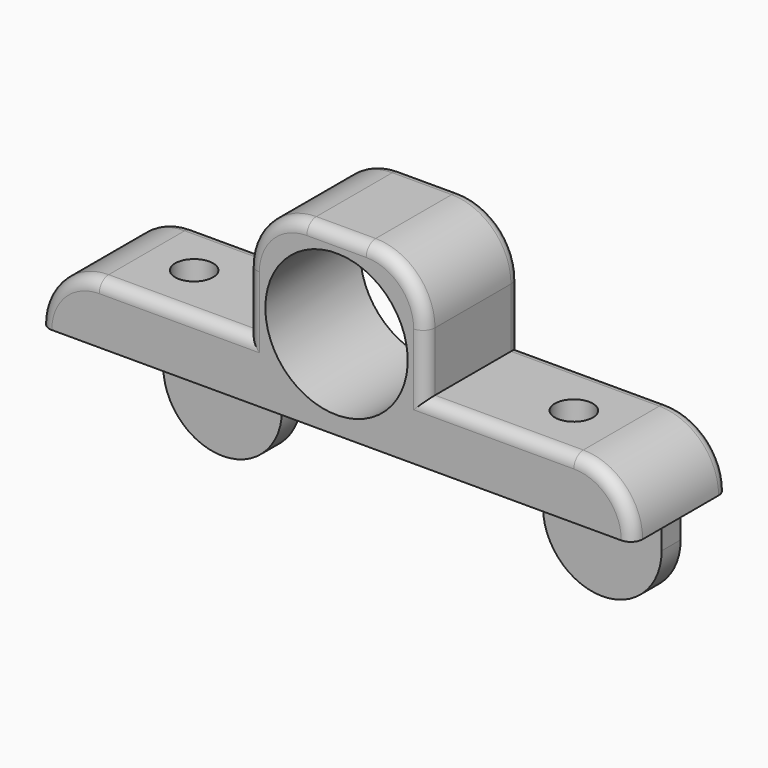
from build123d import *

# Parameters (mm, degrees)
F0_W         = 50
F0_H         = 10
F0_R         = 1.6
F1_DEPTH     = 5
F2_W         = 15
F2_H         = 10
F2_R         = 1.6
F3_DEPTH     = 10
F5_R         = 5
F6_R         = 4.99999
F4_R         = 6
F7_DEPTH     = 25
F8_T1_DEPTH  = 12.50001
F8_T3_DEPTH  = 5
F8_T5_DEPTH  = 5
F8_T7_DEPTH  = 12.50001
F8_T9_DEPTH  = 2.50001
F8_T12_ANGLE = 90
F8_T14_ANGLE = 90
F8_T16_ANGLE = 90
F8_T18_ANGLE = 90
F8_T20_ANGLE = 90
F8_T22_ANGLE = 90
F8_T24_ANGLE = 90
F8_T26_ANGLE = 90
F8_T31_DEPTH = 7.5
F8_T35_DEPTH = 15.00001
F8_T42_DEPTH = 15.00001
F8_T46_DEPTH = 7.5
F8_T53_DEPTH = 15.00001
F8_T57_DEPTH = 7.5
F8_T64_DEPTH = 7.5
F8_T68_DEPTH = 15.00001
F9_W         = 10
F9_H         = 2
F10_DEPTH    = 10
F11_R        = 4.99999


# Not quite as in the source:
# - a fillet or chamfer that OpenCascade refuses, or shapes differently, is made with other operations: its cross-section is extruded or revolved along the edge and cut away or added
# - a fillet or chamfer is up to 0.001 mm smaller than in the source, because OpenCascade refuses the exact size


with BuildPart() as f1:
    # F0 (on Top) → F1 (new body)
    with BuildSketch(Plane.XY):
        Rectangle(F0_W, F0_H)
        with Locations((-16, 0)):
            Circle(F0_R, mode=Mode.SUBTRACT)
        with Locations((16, 0)):
            Circle(F0_R, mode=Mode.SUBTRACT)
    extrude(amount=F1_DEPTH)

    # F2 (on face) → F3 (join)
    with BuildSketch(Plane.XY.offset(5)):
        Rectangle(F2_W, F2_H)
        with Locations((-3.9, 0)):
            Circle(F2_R, mode=Mode.SUBTRACT)
        with Locations((3.9, 0)):
            Circle(F2_R, mode=Mode.SUBTRACT)
        with Locations((3.9, 0)):
            Circle(F2_R)
        with Locations((-3.9, 0)):
            Circle(F2_R)
    extrude(amount=F3_DEPTH)

    # F5
    f5_edges = [f1.edges().sort_by_distance(p)[0] for p in [
        (7.5, 0, 15),
        (-7.5, 0, 15),
    ]]
    fillet(f5_edges, radius=F5_R)

    # F6 (radius 5 in the source; OpenCascade refuses exactly that, so slightly less here)
    f6_edges = [f1.edges().sort_by_distance(p)[0] for p in [
        (-25, 0, 5),
        (25, 0, 5),
    ]]
    fillet(f6_edges, radius=F6_R)

    # F4 (on face) → F7 (cut)
    with BuildSketch(Plane(origin=(0, 5, 0), x_dir=(-1, 0, 0), z_dir=(0, 1, 0))):
        with Locations((0, 7.5)):
            Circle(F4_R)
    extrude(amount=-F7_DEPTH, mode=Mode.SUBTRACT)

    # F8: fillet of radius 1 on 18 edges, made by hand

    # F8_s2 → F8_t1 (cut)
    with BuildSketch(Plane.YZ.offset(7.5)):
        with BuildLine():
            ThreePointArc((-5, 4), (-4.7071067812, 4.7071067812), (-4, 5))
            Line((-4, 5), (-5, 5))
            Line((-5, 5), (-5, 4))
        make_face()
        with BuildLine():
            ThreePointArc((4, 5), (4.7071067812, 4.7071067812), (5, 4))
            Line((5, 4), (5, 5))
            Line((5, 5), (4, 5))
        make_face()
    extrude(amount=F8_T1_DEPTH, mode=Mode.SUBTRACT)

    # F8_s4 → F8_t3 (cut)
    with BuildSketch(Plane.XY.offset(5)):
        with BuildLine():
            ThreePointArc((6.5, -5), (7.2071067812, -4.7071067812), (7.5, -4))
            Line((7.5, -4), (7.5, -5))
            Line((7.5, -5), (6.5, -5))
        make_face()
        with BuildLine():
            ThreePointArc((-6.5, -5), (-7.2071067812, -4.7071067812), (-7.5, -4))
            Line((-7.5, -4), (-7.5, -5))
            Line((-7.5, -5), (-6.5, -5))
        make_face()
        with BuildLine():
            ThreePointArc((7.5, 4), (7.2071067812, 4.7071067812), (6.5, 5))
            Line((6.5, 5), (7.5, 5))
            Line((7.5, 5), (7.5, 4))
        make_face()
        with BuildLine():
            ThreePointArc((-7.5, 4), (-7.2071067812, 4.7071067812), (-6.5, 5))
            Line((-6.5, 5), (-7.5, 5))
            Line((-7.5, 5), (-7.5, 4))
        make_face()
    extrude(amount=F8_T3_DEPTH, mode=Mode.SUBTRACT)

    # F8_s6 → F8_t5 (cut)
    with BuildSketch(Plane.YZ.offset(-2.5)):
        with BuildLine():
            ThreePointArc((-5, 14), (-4.7071067812, 14.7071067812), (-4, 15))
            Line((-4, 15), (-5, 15))
            Line((-5, 15), (-5, 14))
        make_face()
        with BuildLine():
            ThreePointArc((4, 15), (4.7071067812, 14.7071067812), (5, 14))
            Line((5, 14), (5, 15))
            Line((5, 15), (4, 15))
        make_face()
    extrude(amount=F8_T5_DEPTH, mode=Mode.SUBTRACT)

    # F8_s8 → F8_t7 (cut)
    with BuildSketch(Plane.YZ.offset(-20.00001)):
        with BuildLine():
            ThreePointArc((-5, 4), (-4.7071067812, 4.7071067812), (-4, 5))
            Line((-4, 5), (-5, 5))
            Line((-5, 5), (-5, 4))
        make_face()
        with BuildLine():
            ThreePointArc((4, 5), (4.7071067812, 4.7071067812), (5, 4))
            Line((5, 4), (5, 5))
            Line((5, 5), (4, 5))
        make_face()
    extrude(amount=F8_T7_DEPTH, mode=Mode.SUBTRACT)

    # F8_s10 → F8_t9 (cut)
    with BuildSketch(Plane.XY.offset(-2.5)):
        with BuildLine():
            ThreePointArc((-25, 4), (-24.7071067812, 4.7071067812), (-24, 5))
            Line((-24, 5), (-25, 5))
            Line((-25, 5), (-25, 4))
        make_face()
        with BuildLine():
            ThreePointArc((25, 4), (24.7071067812, 4.7071067812), (24, 5))
            Line((24, 5), (25, 5))
            Line((25, 5), (25, 4))
        make_face()
        with BuildLine():
            ThreePointArc((-24, -5), (-24.7071067812, -4.7071067812), (-25, -4))
            Line((-25, -4), (-25, -5))
            Line((-25, -5), (-24, -5))
        make_face()
        with BuildLine():
            ThreePointArc((24, -5), (24.7071067812, -4.7071067812), (25, -4))
            Line((25, -4), (25, -5))
            Line((25, -5), (24, -5))
        make_face()
    extrude(amount=F8_T9_DEPTH, mode=Mode.SUBTRACT)

    # F8_s11 → F8_t12 (revolve, cut)
    with BuildSketch(Plane.XY.offset(1e-05)):
        with BuildLine():
            ThreePointArc((24, -5), (24.7071067812, -4.7071067812), (25, -4))
            Line((25, -4), (25, -5))
            Line((25, -5), (24, -5))
        make_face()
    revolve(axis=Axis((20.00001, -5, 1e-05), (0, -1, 0)), revolution_arc=F8_T12_ANGLE, mode=Mode.SUBTRACT)

    # F8_s13 → F8_t14 (revolve, cut)
    with BuildSketch(Plane.XY.offset(10)):
        with BuildLine():
            ThreePointArc((6.5, -5), (7.2071067812, -4.7071067812), (7.5, -4))
            Line((7.5, -4), (7.5, -5))
            Line((7.5, -5), (6.5, -5))
        make_face()
    revolve(axis=Axis((2.5, -5, 10), (0, -1, 0)), revolution_arc=F8_T14_ANGLE, mode=Mode.SUBTRACT)

    # F8_s15 → F8_t16 (revolve, cut)
    with BuildSketch(Plane.XY.offset(10)):
        with BuildLine():
            ThreePointArc((-6.5, -5), (-7.2071067812, -4.7071067812), (-7.5, -4))
            Line((-7.5, -4), (-7.5, -5))
            Line((-7.5, -5), (-6.5, -5))
        make_face()
    revolve(axis=Axis((-2.5, -5, 10), (0, 1, 0)), revolution_arc=F8_T16_ANGLE, mode=Mode.SUBTRACT)

    # F8_s17 → F8_t18 (revolve, cut)
    with BuildSketch(Plane.YZ.offset(-20.00001)):
        with BuildLine():
            ThreePointArc((-5, 4), (-4.7071067812, 4.7071067812), (-4, 5))
            Line((-4, 5), (-5, 5))
            Line((-5, 5), (-5, 4))
        make_face()
    revolve(axis=Axis((-20.00001, -5, 1e-05), (0, -1, 0)), revolution_arc=F8_T18_ANGLE, mode=Mode.SUBTRACT)

    # F8_s19 → F8_t20 (revolve, cut)
    with BuildSketch(Plane.XY.offset(10)):
        with BuildLine():
            ThreePointArc((7.5, 4), (7.2071067812, 4.7071067812), (6.5, 5))
            Line((6.5, 5), (7.5, 5))
            Line((7.5, 5), (7.5, 4))
        make_face()
    revolve(axis=Axis((2.5, 5, 10), (0, -1, 0)), revolution_arc=F8_T20_ANGLE, mode=Mode.SUBTRACT)

    # F8_s21 → F8_t22 (revolve, cut)
    with BuildSketch(Plane.XY.offset(1e-05)):
        with BuildLine():
            ThreePointArc((25, 4), (24.7071067812, 4.7071067812), (24, 5))
            Line((24, 5), (25, 5))
            Line((25, 5), (25, 4))
        make_face()
    revolve(axis=Axis((20.00001, 5, 1e-05), (0, -1, 0)), revolution_arc=F8_T22_ANGLE, mode=Mode.SUBTRACT)

    # F8_s23 → F8_t24 (revolve, cut)
    with BuildSketch(Plane.XY.offset(10)):
        with BuildLine():
            ThreePointArc((-7.5, 4), (-7.2071067812, 4.7071067812), (-6.5, 5))
            Line((-6.5, 5), (-7.5, 5))
            Line((-7.5, 5), (-7.5, 4))
        make_face()
    revolve(axis=Axis((-2.5, 5, 10), (0, 1, 0)), revolution_arc=F8_T24_ANGLE, mode=Mode.SUBTRACT)

    # F8_s25 → F8_t26 (revolve, cut)
    with BuildSketch(Plane.YZ.offset(-20.00001)):
        with BuildLine():
            ThreePointArc((4, 5), (4.7071067812, 4.7071067812), (5, 4))
            Line((5, 4), (5, 5))
            Line((5, 5), (4, 5))
        make_face()
    revolve(axis=Axis((-20.00001, 5, 1e-05), (0, -1, 0)), revolution_arc=F8_T26_ANGLE, mode=Mode.SUBTRACT)


with BuildPart() as f8_tool29:
    # F8_s30 → F8_t31 (new body)
    with BuildSketch(Plane.XY.offset(2.5)):
        with BuildLine():
            ThreePointArc((6.5, -5), (7.2071067812, -4.7071067812), (7.5, -4))
            Line((7.5, -4), (7.5, -5))
            Line((7.5, -5), (6.5, -5))
        make_face()
    extrude(amount=F8_T31_DEPTH)

    split(bisect_by=Plane.XY.offset(5), keep=Keep.BOTTOM)


with BuildPart() as f8_tool33:
    # F8_s34 → F8_t35 (new body)
    with BuildSketch(Plane.YZ.offset(5)):
        with BuildLine():
            ThreePointArc((-5, 4), (-4.7071067812, 4.7071067812), (-4, 5))
            Line((-4, 5), (-5, 5))
            Line((-5, 5), (-5, 4))
        make_face()
    extrude(amount=F8_T35_DEPTH)

    split(bisect_by=Plane.YZ.offset(7.5), keep=Keep.BOTTOM)


with BuildPart() as f8_tool29_1:
    add(f8_tool29.part)

    # F8_t37: intersect F8_tool33
    add(f8_tool33.part, mode=Mode.INTERSECT)


with BuildPart() as f1_1:
    add(f1.part)

    # F8_t27: cut F8_tool29
    add(f8_tool29_1.part, mode=Mode.SUBTRACT)


with BuildPart() as f8_tool40:
    # F8_s41 → F8_t42 (new body)
    with BuildSketch(Plane.YZ.offset(-20.00001)):
        with BuildLine():
            ThreePointArc((-5, 4), (-4.7071067812, 4.7071067812), (-4, 5))
            Line((-4, 5), (-5, 5))
            Line((-5, 5), (-5, 4))
        make_face()
    extrude(amount=F8_T42_DEPTH)

    split(bisect_by=Plane.YZ.offset(-7.5), keep=Keep.TOP)


with BuildPart() as f8_tool44:
    # F8_s45 → F8_t46 (new body)
    with BuildSketch(Plane.XY.offset(2.5)):
        with BuildLine():
            ThreePointArc((-6.5, -5), (-7.2071067812, -4.7071067812), (-7.5, -4))
            Line((-7.5, -4), (-7.5, -5))
            Line((-7.5, -5), (-6.5, -5))
        make_face()
    extrude(amount=F8_T46_DEPTH)

    split(bisect_by=Plane.XY.offset(5), keep=Keep.BOTTOM)


with BuildPart() as f8_tool40_1:
    add(f8_tool40.part)

    # F8_t48: intersect F8_tool44
    add(f8_tool44.part, mode=Mode.INTERSECT)


with BuildPart() as f1_2:
    add(f1_1.part)

    # F8_t38: cut F8_tool40
    add(f8_tool40_1.part, mode=Mode.SUBTRACT)


with BuildPart() as f8_tool51:
    # F8_s52 → F8_t53 (new body)
    with BuildSketch(Plane.YZ.offset(-5)):
        with BuildLine():
            ThreePointArc((4, 5), (4.7071067812, 4.7071067812), (5, 4))
            Line((5, 4), (5, 5))
            Line((5, 5), (4, 5))
        make_face()
    extrude(amount=-F8_T53_DEPTH)

    split(bisect_by=Plane.YZ.offset(-7.5), keep=Keep.TOP)


with BuildPart() as f8_tool55:
    # F8_s56 → F8_t57 (new body)
    with BuildSketch(Plane.XY.offset(2.5)):
        with BuildLine():
            ThreePointArc((-7.5, 4), (-7.2071067812, 4.7071067812), (-6.5, 5))
            Line((-6.5, 5), (-7.5, 5))
            Line((-7.5, 5), (-7.5, 4))
        make_face()
    extrude(amount=F8_T57_DEPTH)

    split(bisect_by=Plane.XY.offset(5), keep=Keep.BOTTOM)


with BuildPart() as f8_tool51_1:
    add(f8_tool51.part)

    # F8_t59: intersect F8_tool55
    add(f8_tool55.part, mode=Mode.INTERSECT)


with BuildPart() as f1_3:
    add(f1_2.part)

    # F8_t49: cut F8_tool51
    add(f8_tool51_1.part, mode=Mode.SUBTRACT)


with BuildPart() as f8_tool62:
    # F8_s63 → F8_t64 (new body)
    with BuildSketch(Plane.XY.offset(2.5)):
        with BuildLine():
            ThreePointArc((7.5, 4), (7.2071067812, 4.7071067812), (6.5, 5))
            Line((6.5, 5), (7.5, 5))
            Line((7.5, 5), (7.5, 4))
        make_face()
    extrude(amount=F8_T64_DEPTH)

    split(bisect_by=Plane.XY.offset(5), keep=Keep.BOTTOM)


with BuildPart() as f8_tool66:
    # F8_s67 → F8_t68 (new body)
    with BuildSketch(Plane.YZ.offset(20.00001)):
        with BuildLine():
            ThreePointArc((4, 5), (4.7071067812, 4.7071067812), (5, 4))
            Line((5, 4), (5, 5))
            Line((5, 5), (4, 5))
        make_face()
    extrude(amount=-F8_T68_DEPTH)

    split(bisect_by=Plane.YZ.offset(7.5), keep=Keep.BOTTOM)


with BuildPart() as f8_tool62_1:
    add(f8_tool62.part)

    # F8_t70: intersect F8_tool66
    add(f8_tool66.part, mode=Mode.INTERSECT)


with BuildPart() as f1_4:
    add(f1_3.part)

    # F8_t60: cut F8_tool62
    add(f8_tool62_1.part, mode=Mode.SUBTRACT)

    # F9 (on face) → F10 (join)
    with BuildSketch(Plane(origin=(0, 0, 0), x_dir=(1, 0, 0), z_dir=(0, 0, -1))):
        with Locations((-16, -4)):
            Rectangle(F9_W, F9_H)
        with Locations((16, -4)):
            Rectangle(F9_W, F9_H)
    extrude(amount=F10_DEPTH)

    # F11 (radius 5 in the source; OpenCascade refuses exactly that, so slightly less here)
    f11_edges = [f1_4.edges().sort_by_distance(p)[0] for p in [
        (11, 4, -10),
        (21, 4, -10),
        (-21, 4, -10),
        (-11, 4, -10),
    ]]
    fillet(f11_edges, radius=F11_R)


solid = f1_4.part
